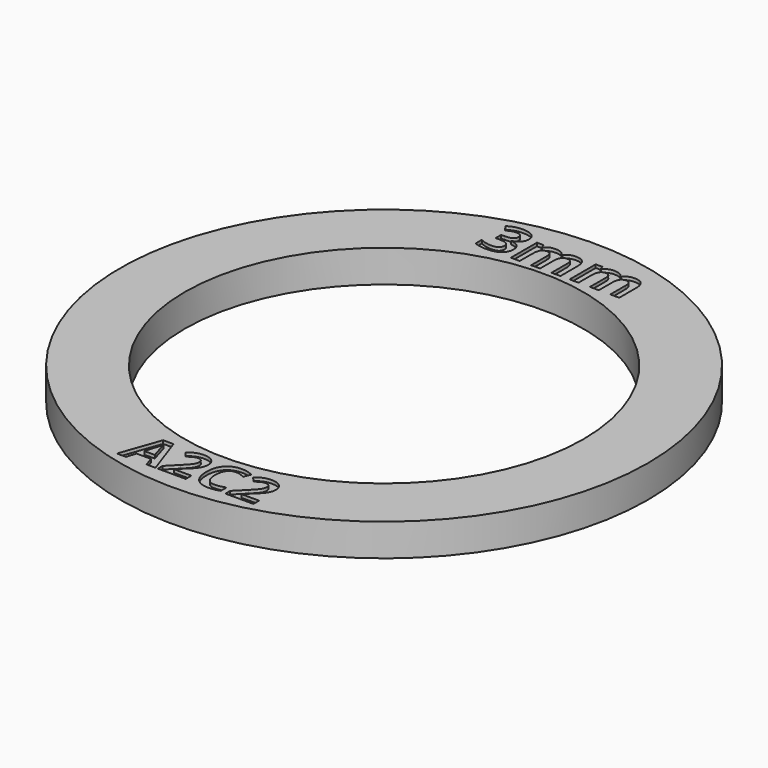
from build123d import *

# Parameters (mm, degrees)
F0_R           = 24.5
F0_R_2         = 18.5
F0_TEXT_SIZE   = 5.1974965673
F0_TEXT_SIZE_2 = 5.5555555556
F1_DEPTH       = 3
F2_DEPTH       = 0.3


# Not quite as in the source:
# - Text() gives the source's letters only with a copy of the font that has no kerning and outlines rounded to 1/6400 em; it was checked with that copy


with BuildPart() as f1:
    # F0 (on Top) → F1 (new body)
    with BuildSketch(Plane.XY):
        Circle(F0_R)
        Polygon((-2.9154707307, -22.8730905801), (-3.7633123583, -22.8730905801), (-4.0321203839, -21.9895161637), (-5.3850937091, -21.9895161637), (-5.6539017347, -22.8730905801), (-6.5017433622, -22.8730905801), (-5.1918118055, -19.1471352284), (-4.2302749405, -19.1471352284), align=None, mode=Mode.SUBTRACT)
        with BuildLine():
            Line((-0.1136952374, -22.2128460943), (-0.1136952374, -22.8730905801))
            Line((-0.1136952374, -22.8730905801), (-2.707570868, -22.8730905801))
            Line((-2.707570868, -22.8730905801), (-2.707570868, -22.3273534405))
            Line((-2.707570868, -22.3273534405), (-1.7760820301, -21.3861192965))
            add(Edge.make_bspline(
                [(-1.7760820301, -21.3861192965), (-1.3619065224, -20.9621984828), (-1.2352175436, -20.7985585518)],
                knots=[0, 0, 0, 1, 1, 1], degree=2))
            add(Edge.make_bspline(
                [(-1.2352175436, -20.7985585518), (-1.1085285648, -20.6349186208), (-1.0524930549, -20.4952359005)],
                knots=[0, 0, 0, 1, 1, 1], degree=2))
            add(Edge.make_bspline(
                [(-1.0524930549, -20.4952359005), (-0.996457545, -20.3555531803), (-0.996457545, -20.206125154)],
                knots=[0, 0, 0, 1, 1, 1], degree=2))
            add(Edge.make_bspline(
                [(-0.996457545, -20.206125154), (-0.996457545, -19.9827952234), (-1.1198980885, -19.8735665846)],
                knots=[0, 0, 0, 1, 1, 1], degree=2))
            add(Edge.make_bspline(
                [(-1.1198980885, -19.8735665846), (-1.243338632, -19.7643379458), (-1.4488021681, -19.7643379458)],
                knots=[0, 0, 0, 1, 1, 1], degree=2))
            add(Edge.make_bspline(
                [(-1.4488021681, -19.7643379458), (-1.6640110104, -19.7643379458), (-1.86703822, -19.8634152241)],
                knots=[0, 0, 0, 1, 1, 1], degree=2))
            add(Edge.make_bspline(
                [(-1.86703822, -19.8634152241), (-2.0700654297, -19.9624925024), (-2.2909590338, -20.1452169911)],
                knots=[0, 0, 0, 1, 1, 1], degree=2))
            Line((-2.2909590338, -20.1452169911), (-2.7173161741, -19.6400852935))
            add(Edge.make_bspline(
                [(-2.7173161741, -19.6400852935), (-2.4436354955, -19.4061979479), (-2.2633473333, -19.3099630505)],
                knots=[0, 0, 0, 1, 1, 1], degree=2))
            add(Edge.make_bspline(
                [(-2.2633473333, -19.3099630505), (-2.0830591711, -19.2137281532), (-1.869880601, -19.1617531875)],
                knots=[0, 0, 0, 1, 1, 1], degree=2))
            add(Edge.make_bspline(
                [(-1.869880601, -19.1617531875), (-1.6567020308, -19.1097782218), (-1.3927666583, -19.1097782218)],
                knots=[0, 0, 0, 1, 1, 1], degree=2))
            add(Edge.make_bspline(
                [(-1.3927666583, -19.1097782218), (-1.0451840753, -19.1097782218), (-0.7788123763, -19.2364672006)],
                knots=[0, 0, 0, 1, 1, 1], degree=2))
            add(Edge.make_bspline(
                [(-0.7788123763, -19.2364672006), (-0.5124406772, -19.3631561795), (-0.365042923, -19.5917648176)],
                knots=[0, 0, 0, 1, 1, 1], degree=2))
            add(Edge.make_bspline(
                [(-0.365042923, -19.5917648176), (-0.2176451688, -19.8203734556), (-0.2176451688, -20.1143568552)],
                knots=[0, 0, 0, 1, 1, 1], degree=2))
            add(Edge.make_bspline(
                [(-0.2176451688, -20.1143568552), (-0.2176451688, -20.3709832482), (-0.3077892498, -20.5955313421)],
                knots=[0, 0, 0, 1, 1, 1], degree=2))
            add(Edge.make_bspline(
                [(-0.3077892498, -20.5955313421), (-0.3979333309, -20.820079436), (-0.5871546903, -21.0559970536)],
                knots=[0, 0, 0, 1, 1, 1], degree=2))
            add(Edge.make_bspline(
                [(-0.5871546903, -21.0559970536), (-0.7763760497, -21.2919146713), (-1.253083938, -21.7288292265)],
                knots=[0, 0, 0, 1, 1, 1], degree=2))
            Line((-1.253083938, -21.7288292265), (-1.7306039352, -22.1779254142))
            Line((-1.7306039352, -22.1779254142), (-1.7306039352, -22.2128460943))
            Line((-1.7306039352, -22.2128460943), (-0.1136952374, -22.2128460943))
        make_face(mode=Mode.SUBTRACT)
        Circle(F0_R_2, mode=Mode.SUBTRACT)
        with BuildLine():
            add(Edge.make_bspline(
                [(2.5077920937, -19.8378337957), (2.2974559045, -19.7643379458), (2.0944286949, -19.7643379458)],
                knots=[0, 0, 0, 1, 1, 1], degree=2))
            add(Edge.make_bspline(
                [(2.0944286949, -19.7643379458), (1.6502051601, -19.7643379458), (1.4065725085, -20.0981146785)],
                knots=[0, 0, 0, 1, 1, 1], degree=2))
            add(Edge.make_bspline(
                [(1.4065725085, -20.0981146785), (1.1629398569, -20.4318914111), (1.1629398569, -21.0279792987)],
                knots=[0, 0, 0, 1, 1, 1], degree=2))
            add(Edge.make_bspline(
                [(1.1629398569, -21.0279792987), (1.1629398569, -22.2688816042), (2.0944286949, -22.2688816042)],
                knots=[0, 0, 0, 1, 1, 1], degree=2))
            add(Edge.make_bspline(
                [(2.0944286949, -22.2688816042), (2.4850530463, -22.2688816042), (3.0405354919, -22.0739754829)],
                knots=[0, 0, 0, 1, 1, 1], degree=2))
            Line((3.0405354919, -22.0739754829), (3.0405354919, -22.7334078599))
            add(Edge.make_bspline(
                [(3.0405354919, -22.7334078599), (2.5841303246, -22.9242534369), (2.0205267906, -22.9242534369)],
                knots=[0, 0, 0, 1, 1, 1], degree=2))
            add(Edge.make_bspline(
                [(2.0205267906, -22.9242534369), (1.2108542784, -22.9242534369), (0.7820608116, -22.4329275896)],
                knots=[0, 0, 0, 1, 1, 1], degree=2))
            add(Edge.make_bspline(
                [(0.7820608116, -22.4329275896), (0.3532673448, -21.9416017422), (0.3532673448, -21.0231066457)],
                knots=[0, 0, 0, 1, 1, 1], degree=2))
            add(Edge.make_bspline(
                [(0.3532673448, -21.0231066457), (0.3532673448, -20.4440730437), (0.5640095884, -20.0087827062)],
                knots=[0, 0, 0, 1, 1, 1], degree=2))
            add(Edge.make_bspline(
                [(0.5640095884, -20.0087827062), (0.7747518321, -19.5734923687), (1.1694367277, -19.3416352953)],
                knots=[0, 0, 0, 1, 1, 1], degree=2))
            add(Edge.make_bspline(
                [(1.1694367277, -19.3416352953), (1.5641216232, -19.1097782218), (2.0944286949, -19.1097782218)],
                knots=[0, 0, 0, 1, 1, 1], degree=2))
            add(Edge.make_bspline(
                [(2.0944286949, -19.1097782218), (2.6344810726, -19.1097782218), (3.1802182121, -19.370465159)],
                knots=[0, 0, 0, 1, 1, 1], degree=2))
            Line((3.1802182121, -19.370465159), (2.9268402545, -20.0104069239))
            add(Edge.make_bspline(
                [(2.9268402545, -20.0104069239), (2.7181282829, -19.9113296456), (2.5077920937, -19.8378337957)],
                knots=[0, 0, 0, 1, 1, 1], degree=2))
        make_face(mode=Mode.SUBTRACT)
        with BuildLine():
            Line((6.1647181942, -22.2128460943), (6.1647181942, -22.8730905801))
            Line((6.1647181942, -22.8730905801), (3.5708425635, -22.8730905801))
            Line((3.5708425635, -22.8730905801), (3.5708425635, -22.3273534405))
            Line((3.5708425635, -22.3273534405), (4.5023314015, -21.3861192965))
            add(Edge.make_bspline(
                [(4.5023314015, -21.3861192965), (4.9165069092, -20.9621984828), (5.043195888, -20.7985585518)],
                knots=[0, 0, 0, 1, 1, 1], degree=2))
            add(Edge.make_bspline(
                [(5.043195888, -20.7985585518), (5.1698848668, -20.6349186208), (5.2259203767, -20.4952359005)],
                knots=[0, 0, 0, 1, 1, 1], degree=2))
            add(Edge.make_bspline(
                [(5.2259203767, -20.4952359005), (5.2819558866, -20.3555531803), (5.2819558866, -20.206125154)],
                knots=[0, 0, 0, 1, 1, 1], degree=2))
            add(Edge.make_bspline(
                [(5.2819558866, -20.206125154), (5.2819558866, -19.9827952234), (5.1585153431, -19.8735665846)],
                knots=[0, 0, 0, 1, 1, 1], degree=2))
            add(Edge.make_bspline(
                [(5.1585153431, -19.8735665846), (5.0350747996, -19.7643379458), (4.8296112634, -19.7643379458)],
                knots=[0, 0, 0, 1, 1, 1], degree=2))
            add(Edge.make_bspline(
                [(4.8296112634, -19.7643379458), (4.6144024212, -19.7643379458), (4.4113752115, -19.8634152241)],
                knots=[0, 0, 0, 1, 1, 1], degree=2))
            add(Edge.make_bspline(
                [(4.4113752115, -19.8634152241), (4.2083480019, -19.9624925024), (3.9874543978, -20.1452169911)],
                knots=[0, 0, 0, 1, 1, 1], degree=2))
            Line((3.9874543978, -20.1452169911), (3.5610972575, -19.6400852935))
            add(Edge.make_bspline(
                [(3.5610972575, -19.6400852935), (3.8347779361, -19.4061979479), (4.0150660983, -19.3099630505)],
                knots=[0, 0, 0, 1, 1, 1], degree=2))
            add(Edge.make_bspline(
                [(4.0150660983, -19.3099630505), (4.1953542604, -19.2137281532), (4.4085328306, -19.1617531875)],
                knots=[0, 0, 0, 1, 1, 1], degree=2))
            add(Edge.make_bspline(
                [(4.4085328306, -19.1617531875), (4.6217114007, -19.1097782218), (4.8856467733, -19.1097782218)],
                knots=[0, 0, 0, 1, 1, 1], degree=2))
            add(Edge.make_bspline(
                [(4.8856467733, -19.1097782218), (5.2332293562, -19.1097782218), (5.4996010553, -19.2364672006)],
                knots=[0, 0, 0, 1, 1, 1], degree=2))
            add(Edge.make_bspline(
                [(5.4996010553, -19.2364672006), (5.7659727544, -19.3631561795), (5.9133705086, -19.5917648176)],
                knots=[0, 0, 0, 1, 1, 1], degree=2))
            add(Edge.make_bspline(
                [(5.9133705086, -19.5917648176), (6.0607682628, -19.8203734556), (6.0607682628, -20.1143568552)],
                knots=[0, 0, 0, 1, 1, 1], degree=2))
            add(Edge.make_bspline(
                [(6.0607682628, -20.1143568552), (6.0607682628, -20.3709832482), (5.9706241817, -20.5955313421)],
                knots=[0, 0, 0, 1, 1, 1], degree=2))
            add(Edge.make_bspline(
                [(5.9706241817, -20.5955313421), (5.8804801006, -20.820079436), (5.6912587412, -21.0559970536)],
                knots=[0, 0, 0, 1, 1, 1], degree=2))
            add(Edge.make_bspline(
                [(5.6912587412, -21.0559970536), (5.5020373818, -21.2919146713), (5.0253294935, -21.7288292265)],
                knots=[0, 0, 0, 1, 1, 1], degree=2))
            Line((5.0253294935, -21.7288292265), (4.5478094964, -22.1779254142))
            Line((4.5478094964, -22.1779254142), (4.5478094964, -22.2128460943))
            Line((4.5478094964, -22.2128460943), (6.1647181942, -22.2128460943))
        make_face(mode=Mode.SUBTRACT)
        with BuildLine():
            add(Edge.make_bspline(
                [(-4.5295138889, 22.7362770999), (-4.1727430556, 22.4867111277), (-4.1727430556, 22.0422666832)],
                knots=[0, 0, 0, 1, 1, 1], degree=2))
            add(Edge.make_bspline(
                [(-4.1727430556, 22.0422666832), (-4.1727430556, 21.6707389055), (-4.3980034722, 21.4103222388)],
                knots=[0, 0, 0, 1, 1, 1], degree=2))
            add(Edge.make_bspline(
                [(-4.3980034722, 21.4103222388), (-4.6232638889, 21.1499055721), (-5.0303819444, 21.0518152944)],
                knots=[0, 0, 0, 1, 1, 1], degree=2))
            Line((-5.0303819444, 21.0518152944), (-5.0303819444, 21.0361902944))
            add(Edge.make_bspline(
                [(-5.0303819444, 21.0361902944), (-4.5494791667, 20.976294461), (-4.3029513889, 20.7440895999)],
                knots=[0, 0, 0, 1, 1, 1], degree=2))
            add(Edge.make_bspline(
                [(-4.3029513889, 20.7440895999), (-4.0564236111, 20.5118847388), (-4.0564236111, 20.1186555721)],
                knots=[0, 0, 0, 1, 1, 1], degree=2))
            add(Edge.make_bspline(
                [(-4.0564236111, 20.1186555721), (-4.0564236111, 19.546606961), (-4.4713541667, 19.2275965444)],
                knots=[0, 0, 0, 1, 1, 1], degree=2))
            add(Edge.make_bspline(
                [(-4.4713541667, 19.2275965444), (-4.8862847222, 18.9085861277), (-5.65625, 18.9085861277)],
                knots=[0, 0, 0, 1, 1, 1], degree=2))
            add(Edge.make_bspline(
                [(-5.65625, 18.9085861277), (-6.3020833333, 18.9085861277), (-6.8012152778, 19.1229958499)],
                knots=[0, 0, 0, 1, 1, 1], degree=2))
            Line((-6.8012152778, 19.1229958499), (-6.8012152778, 19.8365375166))
            add(Edge.make_bspline(
                [(-6.8012152778, 19.8365375166), (-6.5711805556, 19.7202180721), (-6.2942708333, 19.6468673777)],
                knots=[0, 0, 0, 1, 1, 1], degree=2))
            add(Edge.make_bspline(
                [(-6.2942708333, 19.6468673777), (-6.0173611111, 19.5735166832), (-5.7465277778, 19.5735166832)],
                knots=[0, 0, 0, 1, 1, 1], degree=2))
            add(Edge.make_bspline(
                [(-5.7465277778, 19.5735166832), (-5.3307291667, 19.5735166832), (-5.1328125, 19.714575711)],
                knots=[0, 0, 0, 1, 1, 1], degree=2))
            add(Edge.make_bspline(
                [(-5.1328125, 19.714575711), (-4.9348958333, 19.8556347388), (-4.9348958333, 20.1681347388)],
                knots=[0, 0, 0, 1, 1, 1], degree=2))
            add(Edge.make_bspline(
                [(-4.9348958333, 20.1681347388), (-4.9348958333, 20.4467805721), (-5.1627604167, 20.5635340444)],
                knots=[0, 0, 0, 1, 1, 1], degree=2))
            add(Edge.make_bspline(
                [(-5.1627604167, 20.5635340444), (-5.390625, 20.6802875166), (-5.8897569444, 20.6802875166)],
                knots=[0, 0, 0, 1, 1, 1], degree=2))
            Line((-5.8897569444, 20.6802875166), (-6.1909722222, 20.6802875166))
            Line((-6.1909722222, 20.6802875166), (-6.1909722222, 21.3235166832))
            Line((-6.1909722222, 21.3235166832), (-5.8845486111, 21.3235166832))
            add(Edge.make_bspline(
                [(-5.8845486111, 21.3235166832), (-5.4236111111, 21.3235166832), (-5.2105034722, 21.4441764055)],
                knots=[0, 0, 0, 1, 1, 1], degree=2))
            add(Edge.make_bspline(
                [(-5.2105034722, 21.4441764055), (-4.9973958333, 21.5648361277), (-4.9973958333, 21.8573708499)],
                knots=[0, 0, 0, 1, 1, 1], degree=2))
            add(Edge.make_bspline(
                [(-4.9973958333, 21.8573708499), (-4.9973958333, 22.3078916832), (-5.5616319444, 22.3078916832)],
                knots=[0, 0, 0, 1, 1, 1], degree=2))
            add(Edge.make_bspline(
                [(-5.5616319444, 22.3078916832), (-5.7569444444, 22.3078916832), (-5.9592013889, 22.2427875166)],
                knots=[0, 0, 0, 1, 1, 1], degree=2))
            add(Edge.make_bspline(
                [(-5.9592013889, 22.2427875166), (-6.1614583333, 22.1776833499), (-6.4079861111, 22.0179611277)],
                knots=[0, 0, 0, 1, 1, 1], degree=2))
            Line((-6.4079861111, 22.0179611277), (-6.7960069444, 22.5952180721))
            add(Edge.make_bspline(
                [(-6.7960069444, 22.5952180721), (-6.2534722222, 22.9858430721), (-5.5017361111, 22.9858430721)],
                knots=[0, 0, 0, 1, 1, 1], degree=2))
            add(Edge.make_bspline(
                [(-5.5017361111, 22.9858430721), (-4.8862847222, 22.9858430721), (-4.5295138889, 22.7362770999)],
                knots=[0, 0, 0, 1, 1, 1], degree=2))
        make_face(mode=Mode.SUBTRACT)
        with BuildLine():
            Line((-0.6927083333, 20.4849750166), (-0.6927083333, 18.9632736277))
            Line((-0.6927083333, 18.9632736277), (-1.5199652778, 18.9632736277))
            Line((-1.5199652778, 18.9632736277), (-1.5199652778, 20.7349750166))
            add(Edge.make_bspline(
                [(-1.5199652778, 20.7349750166), (-1.5199652778, 21.0631000166), (-1.6297743056, 21.2271625166)],
                knots=[0, 0, 0, 1, 1, 1], degree=2))
            add(Edge.make_bspline(
                [(-1.6297743056, 21.2271625166), (-1.7395833333, 21.3912250166), (-1.9756944444, 21.3912250166)],
                knots=[0, 0, 0, 1, 1, 1], degree=2))
            add(Edge.make_bspline(
                [(-1.9756944444, 21.3912250166), (-2.2934027778, 21.3912250166), (-2.4370659722, 21.1577180721)],
                knots=[0, 0, 0, 1, 1, 1], degree=2))
            add(Edge.make_bspline(
                [(-2.4370659722, 21.1577180721), (-2.5807291667, 20.9242111277), (-2.5807291667, 20.390356961)],
                knots=[0, 0, 0, 1, 1, 1], degree=2))
            Line((-2.5807291667, 20.390356961), (-2.5807291667, 18.9632736277))
            Line((-2.5807291667, 18.9632736277), (-3.4079861111, 18.9632736277))
            Line((-3.4079861111, 18.9632736277), (-3.4079861111, 21.9962597388))
            Line((-3.4079861111, 21.9962597388), (-2.7760416667, 21.9962597388))
            Line((-2.7760416667, 21.9962597388), (-2.6649305556, 21.6082389055))
            Line((-2.6649305556, 21.6082389055), (-2.6189236111, 21.6082389055))
            add(Edge.make_bspline(
                [(-2.6189236111, 21.6082389055), (-2.4965277778, 21.8174402944), (-2.2660590278, 21.9350618221)],
                knots=[0, 0, 0, 1, 1, 1], degree=2))
            add(Edge.make_bspline(
                [(-2.2660590278, 21.9350618221), (-2.0355902778, 22.0526833499), (-1.7369791667, 22.0526833499)],
                knots=[0, 0, 0, 1, 1, 1], degree=2))
            add(Edge.make_bspline(
                [(-1.7369791667, 22.0526833499), (-1.0564236111, 22.0526833499), (-0.8142361111, 21.6082389055)],
                knots=[0, 0, 0, 1, 1, 1], degree=2))
            Line((-0.8142361111, 21.6082389055), (-0.7413194444, 21.6082389055))
            add(Edge.make_bspline(
                [(-0.7413194444, 21.6082389055), (-0.6189236111, 21.820044461), (-0.3819444444, 21.9363639055)],
                knots=[0, 0, 0, 1, 1, 1], degree=2))
            add(Edge.make_bspline(
                [(-0.3819444444, 21.9363639055), (-0.1449652778, 22.0526833499), (0.1536458333, 22.0526833499)],
                knots=[0, 0, 0, 1, 1, 1], degree=2))
            add(Edge.make_bspline(
                [(0.1536458333, 22.0526833499), (0.6692708333, 22.0526833499), (0.93359375, 21.7883604332)],
                knots=[0, 0, 0, 1, 1, 1], degree=2))
            add(Edge.make_bspline(
                [(0.93359375, 21.7883604332), (1.1979166667, 21.5240375166), (1.1979166667, 20.9407041832)],
                knots=[0, 0, 0, 1, 1, 1], degree=2))
            Line((1.1979166667, 20.9407041832), (1.1979166667, 18.9632736277))
            Line((1.1979166667, 18.9632736277), (0.3680555556, 18.9632736277))
            Line((0.3680555556, 18.9632736277), (0.3680555556, 20.7349750166))
            add(Edge.make_bspline(
                [(0.3680555556, 20.7349750166), (0.3680555556, 21.0631000166), (0.2582465278, 21.2271625166)],
                knots=[0, 0, 0, 1, 1, 1], degree=2))
            add(Edge.make_bspline(
                [(0.2582465278, 21.2271625166), (0.1484375, 21.3912250166), (-0.0876736111, 21.3912250166)],
                knots=[0, 0, 0, 1, 1, 1], degree=2))
            add(Edge.make_bspline(
                [(-0.0876736111, 21.3912250166), (-0.3914930556, 21.3912250166), (-0.5421006944, 21.1742111277)],
                knots=[0, 0, 0, 1, 1, 1], degree=2))
            add(Edge.make_bspline(
                [(-0.5421006944, 21.1742111277), (-0.6927083333, 20.9571972388), (-0.6927083333, 20.4849750166)],
                knots=[0, 0, 0, 1, 1, 1], degree=2))
        make_face(mode=Mode.SUBTRACT)
        with BuildLine():
            Line((4.7621527778, 20.4849750166), (4.7621527778, 18.9632736277))
            Line((4.7621527778, 18.9632736277), (3.9348958333, 18.9632736277))
            Line((3.9348958333, 18.9632736277), (3.9348958333, 20.7349750166))
            add(Edge.make_bspline(
                [(3.9348958333, 20.7349750166), (3.9348958333, 21.0631000166), (3.8250868056, 21.2271625166)],
                knots=[0, 0, 0, 1, 1, 1], degree=2))
            add(Edge.make_bspline(
                [(3.8250868056, 21.2271625166), (3.7152777778, 21.3912250166), (3.4791666667, 21.3912250166)],
                knots=[0, 0, 0, 1, 1, 1], degree=2))
            add(Edge.make_bspline(
                [(3.4791666667, 21.3912250166), (3.1614583333, 21.3912250166), (3.0177951389, 21.1577180721)],
                knots=[0, 0, 0, 1, 1, 1], degree=2))
            add(Edge.make_bspline(
                [(3.0177951389, 21.1577180721), (2.8741319444, 20.9242111277), (2.8741319444, 20.390356961)],
                knots=[0, 0, 0, 1, 1, 1], degree=2))
            Line((2.8741319444, 20.390356961), (2.8741319444, 18.9632736277))
            Line((2.8741319444, 18.9632736277), (2.046875, 18.9632736277))
            Line((2.046875, 18.9632736277), (2.046875, 21.9962597388))
            Line((2.046875, 21.9962597388), (2.6788194444, 21.9962597388))
            Line((2.6788194444, 21.9962597388), (2.7899305556, 21.6082389055))
            Line((2.7899305556, 21.6082389055), (2.8359375, 21.6082389055))
            add(Edge.make_bspline(
                [(2.8359375, 21.6082389055), (2.9583333333, 21.8174402944), (3.1888020833, 21.9350618221)],
                knots=[0, 0, 0, 1, 1, 1], degree=2))
            add(Edge.make_bspline(
                [(3.1888020833, 21.9350618221), (3.4192708333, 22.0526833499), (3.7178819444, 22.0526833499)],
                knots=[0, 0, 0, 1, 1, 1], degree=2))
            add(Edge.make_bspline(
                [(3.7178819444, 22.0526833499), (4.3984375, 22.0526833499), (4.640625, 21.6082389055)],
                knots=[0, 0, 0, 1, 1, 1], degree=2))
            Line((4.640625, 21.6082389055), (4.7135416667, 21.6082389055))
            add(Edge.make_bspline(
                [(4.7135416667, 21.6082389055), (4.8359375, 21.820044461), (5.0729166667, 21.9363639055)],
                knots=[0, 0, 0, 1, 1, 1], degree=2))
            add(Edge.make_bspline(
                [(5.0729166667, 21.9363639055), (5.3098958333, 22.0526833499), (5.6085069444, 22.0526833499)],
                knots=[0, 0, 0, 1, 1, 1], degree=2))
            add(Edge.make_bspline(
                [(5.6085069444, 22.0526833499), (6.1241319444, 22.0526833499), (6.3884548611, 21.7883604332)],
                knots=[0, 0, 0, 1, 1, 1], degree=2))
            add(Edge.make_bspline(
                [(6.3884548611, 21.7883604332), (6.6527777778, 21.5240375166), (6.6527777778, 20.9407041832)],
                knots=[0, 0, 0, 1, 1, 1], degree=2))
            Line((6.6527777778, 20.9407041832), (6.6527777778, 18.9632736277))
            Line((6.6527777778, 18.9632736277), (5.8229166667, 18.9632736277))
            Line((5.8229166667, 18.9632736277), (5.8229166667, 20.7349750166))
            add(Edge.make_bspline(
                [(5.8229166667, 20.7349750166), (5.8229166667, 21.0631000166), (5.7131076389, 21.2271625166)],
                knots=[0, 0, 0, 1, 1, 1], degree=2))
            add(Edge.make_bspline(
                [(5.7131076389, 21.2271625166), (5.6032986111, 21.3912250166), (5.3671875, 21.3912250166)],
                knots=[0, 0, 0, 1, 1, 1], degree=2))
            add(Edge.make_bspline(
                [(5.3671875, 21.3912250166), (5.0633680556, 21.3912250166), (4.9127604167, 21.1742111277)],
                knots=[0, 0, 0, 1, 1, 1], degree=2))
            add(Edge.make_bspline(
                [(4.9127604167, 21.1742111277), (4.7621527778, 20.9571972388), (4.7621527778, 20.4849750166)],
                knots=[0, 0, 0, 1, 1, 1], degree=2))
        make_face(mode=Mode.SUBTRACT)
        with BuildLine():
            Line((-5.1869391524, -21.3300837867), (-4.2205296344, -21.3300837867))
            add(Edge.make_bspline(
                [(-4.2205296344, -21.3300837867), (-4.5932875914, -20.1297869232), (-4.640389904, -19.9722378085)],
                knots=[0, 0, 0, 1, 1, 1], degree=2))
            add(Edge.make_bspline(
                [(-4.640389904, -19.9722378085), (-4.6874922167, -19.8146886938), (-4.7077949376, -19.7237325038)],
                knots=[0, 0, 0, 1, 1, 1], degree=2))
            add(Edge.make_bspline(
                [(-4.7077949376, -19.7237325038), (-4.791442148, -20.0485760393), (-5.1869391524, -21.3300837867)],
                knots=[0, 0, 0, 1, 1, 1], degree=2))
        make_face()
        with Locations((-6.5017433622, -22.8730905801)):
            Text('A2C2', F0_TEXT_SIZE, font='Open Sans', font_style=FontStyle.BOLD, text_align=(TextAlign.LEFT, TextAlign.BOTTOM))
        with Locations((-7.0130208333, 18.9632736277)):
            Text('3mm', F0_TEXT_SIZE_2, font='Open Sans', font_style=FontStyle.BOLD, text_align=(TextAlign.LEFT, TextAlign.BOTTOM))
    extrude(amount=-F1_DEPTH)

    # F0 (on Top) → F2 (cut)
    with BuildSketch(Plane.XY):
        with Locations((-6.5017433622, -22.8730905801)):
            Text('A2C2', F0_TEXT_SIZE, font='Open Sans', font_style=FontStyle.BOLD, text_align=(TextAlign.LEFT, TextAlign.BOTTOM))
        with Locations((-7.0130208333, 18.9632736277)):
            Text('3mm', F0_TEXT_SIZE_2, font='Open Sans', font_style=FontStyle.BOLD, text_align=(TextAlign.LEFT, TextAlign.BOTTOM))
    extrude(amount=-F2_DEPTH, mode=Mode.SUBTRACT)


solid = f1.part
